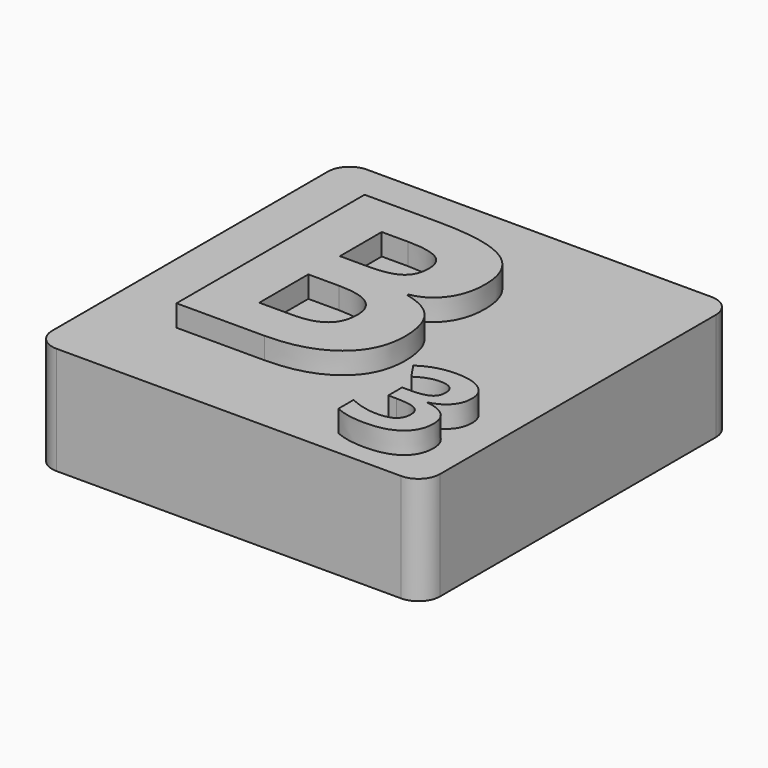
from build123d import *

# Parameters (mm, degrees)
F0_W           = 18
F0_H           = 18
F1_DEPTH       = 5
F2_W           = 16
F2_H           = 16
F3_DEPTH       = 3
F4_TEXT_SIZE   = 15.2777777778
F4_TEXT_SIZE_2 = 6.9444444444
F5_DEPTH       = 1
F6_R           = 1


# Not quite as in the source:
# - Text() gives the source's letters only with a copy of the font that has no kerning and outlines rounded to 1/6400 em; it was checked with that copy


with BuildPart() as f1:
    # F0 (on Top) → F1 (new body)
    with BuildSketch(Plane.XY):
        with Locations((5.0695089158, -1.7574313941)):
            Rectangle(F0_W, F0_H)
    extrude(amount=F1_DEPTH)

    # F2 (on Top) → F3 (cut)
    with BuildSketch(Plane.XY):
        with Locations((5.0695089158, -1.7574313941)):
            Rectangle(F2_W, F2_H)
    extrude(amount=F3_DEPTH, mode=Mode.SUBTRACT)

    # F4 (on face) → F5 (join)
    with BuildSketch(Plane.XY.offset(5)):
        with Locations((-1.9304910842, -6.7574313941)):
            Text('B', F4_TEXT_SIZE, font='Open Sans', font_style=FontStyle.BOLD, text_align=(TextAlign.LEFT, TextAlign.BOTTOM))
        with Locations((8.9234585685, -9.7574313941)):
            Text('3', F4_TEXT_SIZE_2, font='Open Sans', font_style=FontStyle.BOLD, text_align=(TextAlign.LEFT, TextAlign.BOTTOM))
    extrude(amount=F5_DEPTH)

    # F6
    f6_edges = [f1.edges().sort_by_distance(p)[0] for p in [
        (14.069509, 7.242569, 2.5),
        (14.069509, -10.757431, 2.5),
        (-3.930491, -10.757431, 2.5),
        (-3.930491, 7.242569, 2.5),
        (13.069509, -9.757431, 1.5),
        (-2.930491, -9.757431, 1.5),
        (-2.930491, 6.242569, 1.5),
        (13.069509, 6.242569, 1.5),
    ]]
    fillet(f6_edges, radius=F6_R)


solid = f1.part
